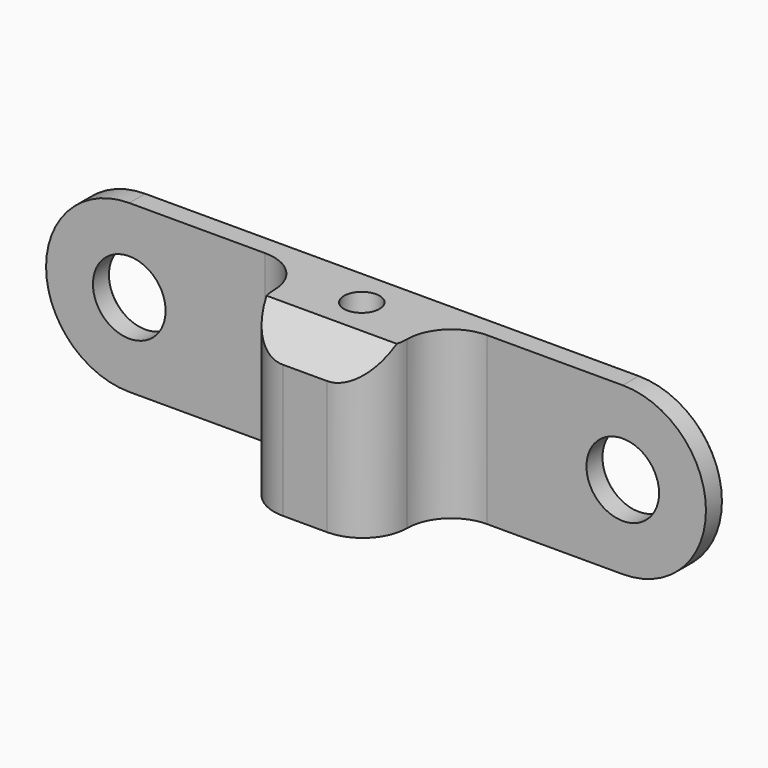
from build123d import *

# Parameters (mm, degrees)
F0_R         = 3.275
F1_DEPTH     = 2
F3_W         = 8
F3_H         = 15
F4_DEPTH     = 6
F5_SIZE      = 3
F6_R         = 3.99999
F8_SIZE      = 0.2
F9_TEXT_SIZE = 17.2508547706
F10_DEPTH    = 0.2


# Not quite as in the source:
# - a fillet or chamfer is up to 0.001 mm smaller than in the source, because OpenCascade refuses the exact size
# - Text() gives the source's letters only with a copy of the font that has no kerning and outlines rounded to 1/6400 em; it was checked with that copy


with BuildPart() as f1:
    # F0 (on Front) → F1 (new body)
    with BuildSketch(Plane.XZ):
        with BuildLine():
            ThreePointArc((-22.25, 7.5), (-29.75, 0), (-22.25, -7.5))
            Line((-22.25, -7.5), (22.25, -7.5))
            ThreePointArc((22.25, -7.5), (29.75, 0), (22.25, 7.5))
            Line((22.25, 7.5), (-22.25, 7.5))
        make_face()
        with Locations((-22.25, 0)):
            Circle(F0_R, mode=Mode.SUBTRACT)
        with Locations((22.25, 0)):
            Circle(F0_R, mode=Mode.SUBTRACT)
    extrude(amount=-F1_DEPTH)

    # F3 (on Right) → F4 (join, symmetric)
    with BuildSketch(Plane.YZ):
        with Locations((-4, 0)):
            Rectangle(F3_W, F3_H)
    extrude(amount=F4_DEPTH, both=True)

    # F5
    f5_edges = [f1.edges().sort_by_distance(p)[0] for p in [
        (0, -8, 7.5),
    ]]
    chamfer(f5_edges, length=F5_SIZE)

    # F6 (radius 4 in the source; OpenCascade refuses exactly that, so slightly less here)
    f6_edges = [f1.edges().sort_by_distance(p)[0] for p in [
        (6, 0, 0),
        (-6, 0, 0),
        (6, -8, -1.5),
        (-6, -8, -1.5),
    ]]
    fillet(f6_edges, radius=F6_R)

    # F2 (on Right) → F7 (revolve, cut)
    with BuildSketch(Plane.YZ):
        Polygon((-4.2336919469, -4.1754380003), (-2.6397804299, -4.3148871887), (1.4032819768, 41.8975275835), (-0.1906295401, 42.0369767719), align=None)
    revolve(axis=Axis((0, -0.6182492266, 18.7913201974), (0, -0.0871557427, -0.9961946981)), mode=Mode.SUBTRACT)

    # F8
    f8_edges = [f1.edges().sort_by_distance(p)[0] for p in [
        (-29.75, 2, 0),
        (0, 2, -7.5),
        (29.75, 2, 0),
        (0, 2, 7.5),
        (-25.525, 2, 0),
        (18.975, 2, 0),
    ]]
    chamfer(f8_edges, length=F8_SIZE)

    # F9 (on face) → F10 (cut)
    with BuildSketch(Plane(origin=(0, 2, 0), x_dir=(-1, 0, 0), z_dir=(0, 1, 0))):
        with Locations((-5.0957407725, -6.2103077174)):
            Text('5', F9_TEXT_SIZE, font='Open Sans', font_style=FontStyle.BOLD, text_align=(TextAlign.LEFT, TextAlign.BOTTOM))
    extrude(amount=-F10_DEPTH, mode=Mode.SUBTRACT)


solid = f1.part
